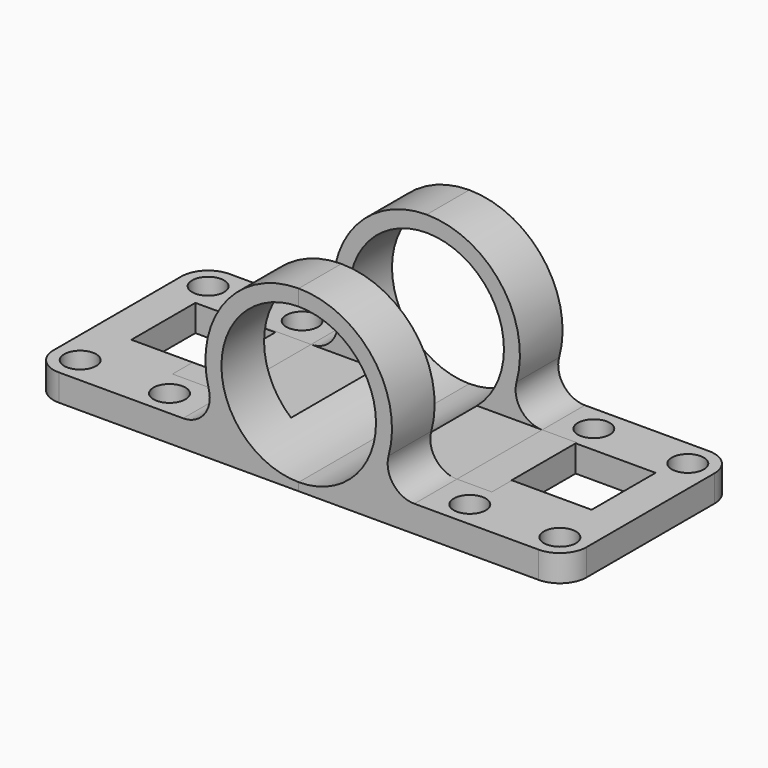
from build123d import *
from build123d import SkipClean  # not in build123d's __all__

# Parameters (mm, degrees)
F0_R      = 14.5
F1_DEPTH  = 40
F2_R      = 5
F3_R      = 5
F4_W      = 15
F4_H      = 15
F4_R      = 3
F5_DEPTH  = 25
F6_W      = 110.2663613856
F6_H      = 71.1540803313
F7_DEPTH  = 50.001
F9_W      = 49.9149149903
F9_H      = 20
F10_DEPTH = 28.501


with BuildPart() as f1:
    # F0 (on Front) → F1 (new body)
    with BuildSketch(Plane.XZ):
        with BuildLine():
            Line((-13.6106575888, -11), (-50, -11))
            Line((-50, -11), (-50, -16))
            Line((-50, -16), (50, -16))
            Line((50, -16), (50, -11))
            Line((50, -11), (13.6106575888, -11))
            ThreePointArc((13.6106575888, -11), (0, 17.5), (-13.6106575888, -11))
        make_face()
        Circle(F0_R, mode=Mode.SUBTRACT)
    extrude(amount=F1_DEPTH)

    # F2
    f2_edges = [f1.edges().sort_by_distance(p)[0] for p in [
        (13.610658, -20, -11),
        (-13.610658, -20, -11),
    ]]
    fillet(f2_edges, radius=F2_R)

    # F3
    f3_edges = [f1.edges().sort_by_distance(p)[0] for p in [
        (50, -40, -13.5),
        (-50, -40, -13.5),
        (50, 0, -13.5),
        (-50, 0, -13.5),
    ]]
    fillet(f3_edges, radius=F3_R)

    # F4 (on face) → F5 (cut)
    with BuildSketch(Plane.XY.offset(-11)):
        with Locations((-35.6688876305, -17.775596238)):
            Rectangle(F4_W, F4_H)
        with Locations((-45, -35)):
            Circle(F4_R)
        with Locations((-28.1688876305, -35.0887903643)):
            Circle(F4_R)
        with Locations((-45, -5)):
            Circle(F4_R)
        with Locations((-27.3576099426, -5)):
            Circle(F4_R)
    extrude(amount=-F5_DEPTH, mode=Mode.SUBTRACT)

    # F6 (on Right) → F7 (cut, through all)
    with BuildSketch(Plane.YZ):
        with Locations((-21.3294159621, -6.3556879759)):
            Rectangle(F6_W, F6_H)
    extrude(amount=F7_DEPTH, mode=Mode.SUBTRACT)

    # F8: F1 across plane


with BuildPart() as f1_1:
    add(f1.part, clean=False)
    with SkipClean():  # cleaning this boolean's faces spoils the solid; the shape is the same uncleaned
        add(f1.part.mirror(Plane.YZ), clean=False)

    # F9 (on face) → F10 (cut, through all)
    with BuildSketch(Plane.XY.offset(-11)):
        Polygon((-21.6852484422, -10), (-31.6722874067, -10), (-31.6722874067, -10.275596238), (-28.1688876305, -10.275596238), (-28.1688876305, -25.275596238), (-31.6722874067, -25.275596238), (-31.6722874067, -30), (-21.6852484422, -30), align=None)
        with Locations((3.272209053, -20)):
            Rectangle(F9_W, F9_H)
    with SkipClean():  # cleaning this boolean's faces spoils the solid; the shape is the same uncleaned
        extrude(amount=F10_DEPTH, mode=Mode.SUBTRACT)


solid = f1_1.part
